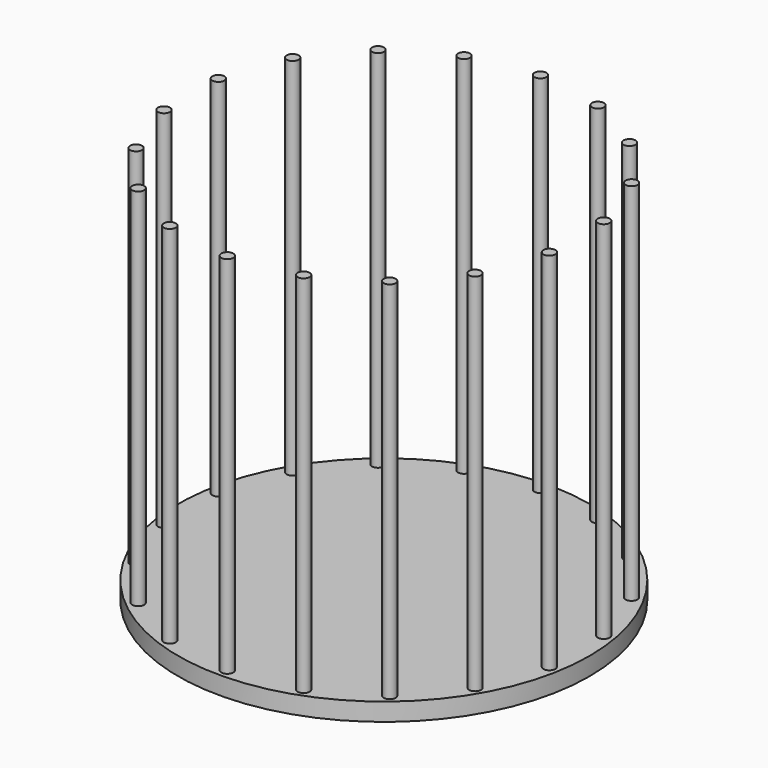
from build123d import *

# Parameters (mm, degrees)
F1_START        = -67.31
F0_R            = 78.74
F1_DEPTH        = 6.858
F2_R            = 2.285444595
F3_DEPTH        = 139.7
F3_COPIES_COUNT = 18


# Not quite as in the source:
# - a pattern or mirror of a feature is missing from the dataset's text; its kind, count and spacing are read off the source's solid


with BuildPart() as f1:
    # F0 (on Top) → F1 (new body)
    with BuildSketch(Plane.XY.offset(F1_START)):
        Circle(F0_R)
    extrude(amount=-F1_DEPTH)

    # F2 (on face) → F3 (join)
    with BuildSketch(Plane.XY.offset(-67.31)):
        with Locations((0, 74.8899579048)):
            Circle(F2_R)
    f3 = extrude(amount=F3_DEPTH)

    # F3_copies: F3 ×18 about axis
    f3_copies_axis = Axis((0, 0, 0), (0, 0, 1))
    for i in range(1, F3_COPIES_COUNT):
        add(f3.rotate(f3_copies_axis, i * 360 / F3_COPIES_COUNT))


solid = f1.part
